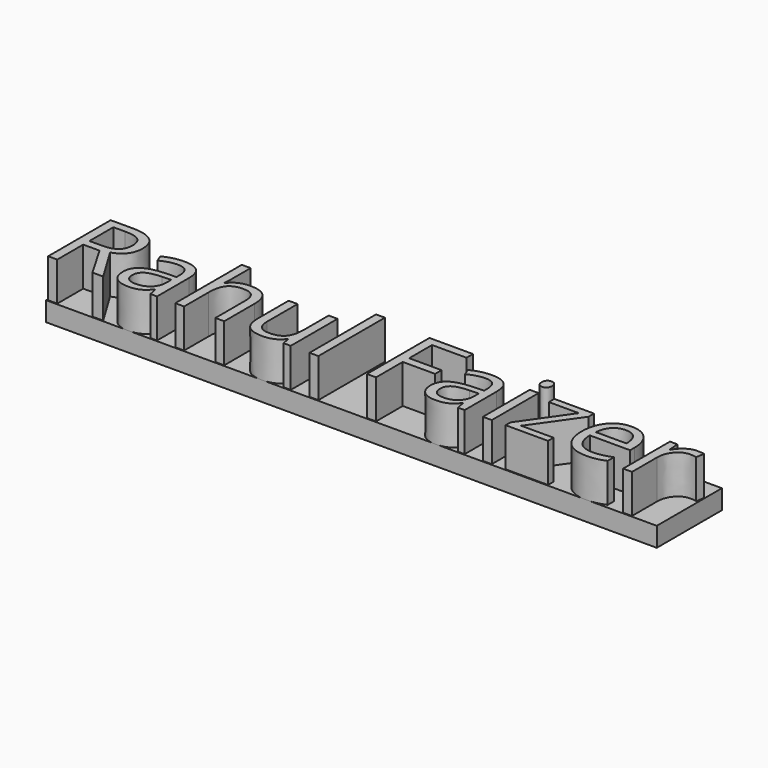
from build123d import *

# Parameters (mm, degrees)
F1_W         = 399.852886796
F1_H         = 53.3090084791
F2_DEPTH     = 12.7
F0_TEXT_SIZE = 71.6151747232
F3_DEPTH     = 25.4


# Not quite as in the source:
# - Text() gives the source's letters only with a copy of the font that has no kerning and outlines rounded to 1/6400 em; it was checked with that copy


with BuildPart() as f2:
    # F1 (on Top) → F2 (new body)
    with BuildSketch(Plane.XY):
        with Locations((1.2138262391, 4.9710273743)):
            Rectangle(F1_W, F1_H)
    extrude(amount=-F2_DEPTH)

    # F0 (on Top) → F3 (join)
    with BuildSketch(Plane.XY):
        with Locations((-204.8446945846, -21.0903212428)):
            Text('Rahul Faizer', F0_TEXT_SIZE, font='Open Sans', text_align=(TextAlign.LEFT, TextAlign.BOTTOM))
    extrude(amount=F3_DEPTH)


solid = f2.part
